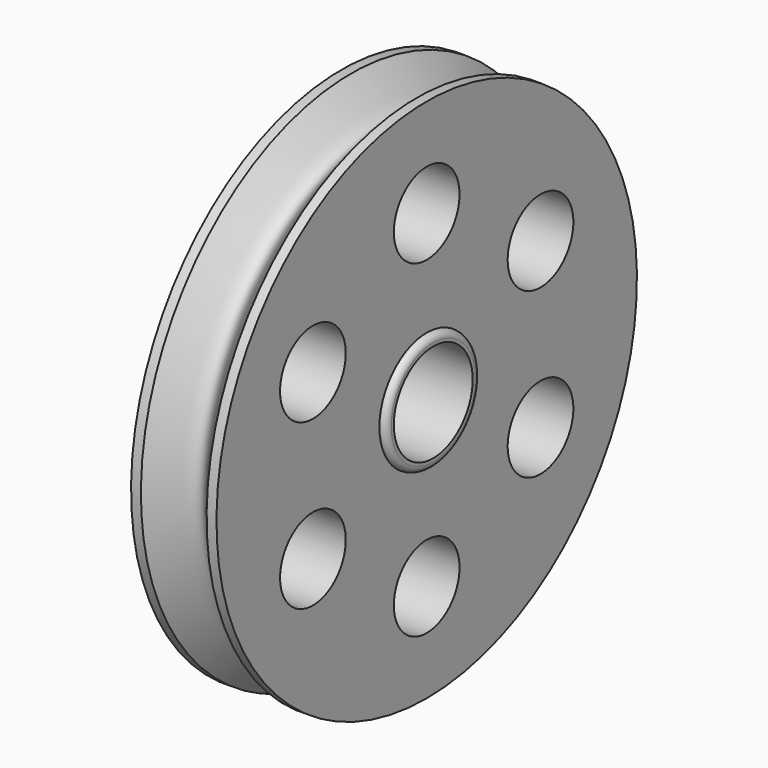
from build123d import *

# Parameters (mm, degrees)
F0_W          = 3
F0_H          = 80
F2_R          = 12.5
F3_DEPTH      = 119.80777
F4_R          = 15
F5_DEPTH      = 102.88035
F4_R_2        = 18
F6_DEPTH      = 2
F6_DEPTH_BACK = 28
F7_R          = 1.99999


# Not quite as in the source:
# - a fillet or chamfer is up to 0.001 mm smaller than in the source, because OpenCascade refuses the exact size


with BuildPart() as f1:
    # F0 (on Front) → F1 (revolve)
    with BuildSketch(Plane.XZ):
        with Locations((11.5, -40)):
            Rectangle(F0_W, F0_H)
        with BuildLine():
            Line((10, -80), (10, 0))
            Line((10, 0), (0, 0))
            Line((0, 0), (-10, 0))
            Line((-10, 0), (-10, -80))
            add(Edge.make_bspline(
                [(-10, -80), (-6, -75.3330111863), (0, -64.6669888505), (6, -75.3330111128), (10, -80)],
                knots=[0, 0, 0, 0, 0.5, 1, 1, 1, 1], degree=3))
        make_face()
        with Locations((-11.5, -40)):
            Rectangle(F0_W, F0_H)
    revolve(axis=Axis((-1.5, 0, 0), (-1, 0, 0)))

    # F2 (on face) → F3 (cut)
    with BuildSketch(Plane(origin=(-13, 0, 0), x_dir=(0, -1, 0), z_dir=(-1, 0, 0))):
        with Locations((-43.3012701892, 25)):
            Circle(F2_R)
        with Locations((43.3012701892, 25)):
            Circle(F2_R)
        with Locations((43.3012701892, -25)):
            Circle(F2_R)
        with Locations((0, -50)):
            Circle(F2_R)
        with Locations((-43.3012701892, -25)):
            Circle(F2_R)
        with Locations((0, 50)):
            Circle(F2_R)
    extrude(amount=-F3_DEPTH, mode=Mode.SUBTRACT)

    # F4 (on face) → F5 (cut)
    with BuildSketch(Plane(origin=(-13, 0, 0), x_dir=(0, -1, 0), z_dir=(-1, 0, 0))):
        Circle(F4_R)
    extrude(amount=-F5_DEPTH, mode=Mode.SUBTRACT)

    # F4 (on face) → F6 (join, two sides)
    with BuildSketch(Plane(origin=(-13, 0, 0), x_dir=(0, -1, 0), z_dir=(-1, 0, 0))) as f6_sk:
        Circle(F4_R_2)
        Circle(F4_R, mode=Mode.SUBTRACT)
    extrude(amount=F6_DEPTH)
    extrude(f6_sk.sketch, amount=-F6_DEPTH_BACK)

    # F7 (radius 2 in the source; OpenCascade refuses exactly that, so slightly less here)
    f7_edges = [f1.edges().sort_by_distance(p)[0] for p in [
        (-15, 18, 0),
        (15, 18, 0),
    ]]
    fillet(f7_edges, radius=F7_R)


solid = f1.part
